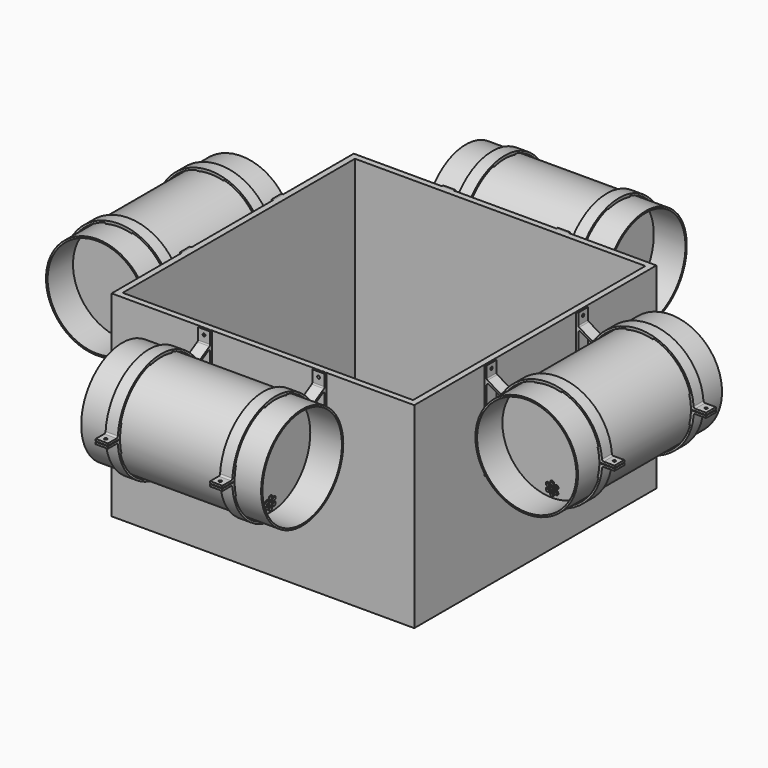
from build123d import *

# Parameters (mm, degrees)
F1_DEPTH    = 139.7
F3_COUNT    = 4
F4_W        = 469.9
F4_H        = 469.9
F4_W_2      = 450.85
F4_H_2      = 450.85
F5_DEPTH    = 304.8
F8_R        = 3.175
F9_DEPTH    = 1.5875
F14_COUNT   = 4
F16_DEPTH   = 9.525
F17_DEPTH   = 9.525
F19_D       = 4.318
F19_DEPTH   = 12.7
F19_TIP     = 1.2972580765
F21_D       = 4.318
F21_DEPTH   = 12.7
F21_TIP     = 1.2972580765
F21_2_D     = 4.318
F21_2_DEPTH = 12.7
F21_2_TIP   = 1.2972580765
F23_COUNT   = 4


with BuildPart() as f1:
    # F0 (on Front) → F1 (new body, symmetric)
    with BuildSketch(Plane.XZ):
        with BuildLine():
            ThreePointArc((413.0675, 228.6), (333.375, 308.2925), (253.6825, 228.6))
            ThreePointArc((253.6825, 228.6), (333.375, 148.9075), (413.0675, 228.6))
        make_face()
        with BuildLine():
            ThreePointArc((410.5275, 228.6), (333.375, 151.4475), (256.2225, 228.6))
            ThreePointArc((256.2225, 228.6), (333.375, 305.7525), (410.5275, 228.6))
        make_face(mode=Mode.SUBTRACT)
    extrude(amount=F1_DEPTH, both=True)


with BuildPart() as f3_1:
    # F3: instance of F1
    add(f1.part.rotate(Axis((0, 0, 60.423810035), (0, 0, 1)), 1 * 360 / F3_COUNT))


with BuildPart() as f3_2:
    # F3: instance of F1
    add(f1.part.rotate(Axis((0, 0, 60.423810035), (0, 0, 1)), 2 * 360 / F3_COUNT))


with BuildPart() as f3_3:
    # F3: instance of F1
    add(f1.part.rotate(Axis((0, 0, 60.423810035), (0, 0, 1)), 3 * 360 / F3_COUNT))


with BuildPart() as f5:
    # F4 (on Top) → F5 (new body)
    with BuildSketch(Plane.XY):
        Rectangle(F4_W, F4_H)
        Rectangle(F4_W_2, F4_H_2, mode=Mode.SUBTRACT)
    extrude(amount=F5_DEPTH)

    # F21 (one way)
    with BuildSketch(Plane.XZ.offset(238.125)):
        with Locations((88.9, 296.855700245), (88.9, 160.344299755)):
            Circle(F21_D / 2)
    extrude(amount=-F21_DEPTH, mode=Mode.SUBTRACT)
    with Locations(Plane.XZ.offset(238.125)):
        with Locations((88.9, 296.855700245), (88.9, 160.344299755)):
            with Locations((0, 0, -(F21_DEPTH + F21_TIP / 2))):  # 118° drill point
                Cone(0, F21_D / 2, F21_TIP, mode=Mode.SUBTRACT)


with BuildPart() as f9:
    # F8 (on Right) → F9 (new body, symmetric)
    with BuildSketch(Plane.YZ):
        with BuildLine():
            ThreePointArc((-333.375, 151.4475), (-278.8199440645, 174.0449440645), (-256.2225, 228.6))
            ThreePointArc((-256.2225, 228.6), (-387.9300559355, 283.1550559355), (-333.375, 151.4475))
        make_face()
        with Locations((-339.9741135768, 160.3375)):
            Circle(F8_R, mode=Mode.SUBTRACT)
        with BuildLine():
            ThreePointArc((-330.2, 156.5275), (-331.1299359697, 154.2824359697), (-333.375, 153.3525))
            ThreePointArc((-333.375, 153.3525), (-336.55, 156.5275), (-333.375, 159.7025))
            ThreePointArc((-333.375, 159.7025), (-331.1299359697, 158.7725640303), (-330.2, 156.5275))
        make_face(mode=Mode.SUBTRACT)
        with BuildLine():
            ThreePointArc((-330.2, 164.1475), (-331.1299359697, 161.9024359697), (-333.375, 160.9725))
            ThreePointArc((-333.375, 160.9725), (-336.55, 164.1475), (-333.375, 167.3225))
            ThreePointArc((-333.375, 167.3225), (-331.1299359697, 166.3925640303), (-330.2, 164.1475))
        make_face(mode=Mode.SUBTRACT)
        with Locations((-339.9741135768, 167.9575)):
            Circle(F8_R, mode=Mode.SUBTRACT)
        with BuildLine():
            ThreePointArc((-330.2, 171.7675), (-331.1299359697, 169.5224359697), (-333.375, 168.5925))
            ThreePointArc((-333.375, 168.5925), (-336.55, 171.7675), (-333.375, 174.9425))
            ThreePointArc((-333.375, 174.9425), (-331.1299359697, 174.0125640303), (-330.2, 171.7675))
        make_face(mode=Mode.SUBTRACT)
        with Locations((-326.7758864232, 160.3375)):
            Circle(F8_R, mode=Mode.SUBTRACT)
        with Locations((-326.7758864232, 167.9575)):
            Circle(F8_R, mode=Mode.SUBTRACT)
    extrude(amount=F9_DEPTH, both=True)


with BuildPart() as f12_1:
    # F12: instance of F9
    add(f9.part.mirror(Plane.YZ.offset(-44.45)))


with BuildPart() as f13_1:
    # F13: instance of F9
    add(f9.part.mirror(Plane.YZ.offset(44.45)))


with BuildPart() as f14_1:
    # F14: instance of F13_1
    add(f13_1.part.rotate(Axis((0, 0, 60.423810035), (0, 0, 1)), 1 * 360 / F14_COUNT))


with BuildPart() as f14_2:
    # F14: instance of F13_1
    add(f13_1.part.rotate(Axis((0, 0, 60.423810035), (0, 0, 1)), 2 * 360 / F14_COUNT))


with BuildPart() as f14_3:
    # F14: instance of F13_1
    add(f13_1.part.rotate(Axis((0, 0, 60.423810035), (0, 0, 1)), 3 * 360 / F14_COUNT))


with BuildPart() as f14_4:
    # F14: instance of F12_1
    add(f12_1.part.rotate(Axis((0, 0, 60.423810035), (0, 0, 1)), 1 * 360 / F14_COUNT))


with BuildPart() as f14_5:
    # F14: instance of F12_1
    add(f12_1.part.rotate(Axis((0, 0, 60.423810035), (0, 0, 1)), 2 * 360 / F14_COUNT))


with BuildPart() as f14_6:
    # F14: instance of F12_1
    add(f12_1.part.rotate(Axis((0, 0, 60.423810035), (0, 0, 1)), 3 * 360 / F14_COUNT))


with BuildPart() as f14_7:
    # F14: instance of F9
    add(f9.part.rotate(Axis((0, 0, 60.423810035), (0, 0, 1)), 1 * 360 / F14_COUNT))


with BuildPart() as f14_8:
    # F14: instance of F9
    add(f9.part.rotate(Axis((0, 0, 60.423810035), (0, 0, 1)), 2 * 360 / F14_COUNT))


with BuildPart() as f14_9:
    # F14: instance of F9
    add(f9.part.rotate(Axis((0, 0, 60.423810035), (0, 0, 1)), 3 * 360 / F14_COUNT))


with BuildPart() as f16:
    # F15 (on offset) → F16 (new body, symmetric)
    with BuildSketch(Plane.YZ.offset(88.9)):
        Polygon((-234.15625, 284.0508849165), (-234.95, 285.425700245), (-234.95, 283.5926131403), align=None)
        Polygon((-234.95, 173.6073868597), (-234.95, 171.774299755), (-234.15625, 173.1491150835), align=None)
        with BuildLine():
            Line((-234.95, 171.774299755), (-260.5097875891, 186.53125))
            ThreePointArc((-260.5097875891, 186.53125), (-261.5323767442, 184.8078044626), (-262.5957219044, 183.1092020457))
            ThreePointArc((-262.5957219044, 183.1092020457), (-261.0577707968, 184.2043074512), (-259.1889889808, 183.9355994633))
            Line((-259.1889889808, 183.9355994633), (-239.395, 172.5075345969))
            ThreePointArc((-239.395, 172.5075345969), (-238.4652954744, 171.5778300713), (-238.125, 170.3078300713))
            Line((-238.125, 170.3078300713), (-238.125, 152.724299755))
            Line((-238.125, 152.724299755), (-234.95, 152.724299755))
            Line((-234.95, 152.724299755), (-234.95, 171.774299755))
        make_face()
        with BuildLine():
            Line((-234.95, 228.6), (-249.2375, 228.6))
            ThreePointArc((-249.2375, 228.6), (-249.2613654173, 226.596157805), (-249.3329481306, 224.593452381))
            ThreePointArc((-249.3329481306, 224.593452381), (-248.5485961043, 226.3108170357), (-246.7958295836, 227.0125))
            Line((-246.7958295836, 227.0125), (-240.665, 227.0125))
            ThreePointArc((-240.665, 227.0125), (-238.8689487758, 226.2685512242), (-238.125, 224.4725))
            Line((-238.125, 224.4725), (-238.125, 179.8398830156))
            ThreePointArc((-238.125, 179.8398830156), (-239.395, 177.64017849), (-241.935, 177.64017849))
            Line((-241.935, 177.64017849), (-257.6014889808, 186.6852301203))
            ThreePointArc((-257.6014889808, 186.6852301203), (-258.7685878325, 188.1692886531), (-258.5891742854, 190.0487460848))
            ThreePointArc((-258.5891742854, 190.0487460848), (-259.5285345493, 188.2785609547), (-260.5097875891, 186.53125))
            Line((-260.5097875891, 186.53125), (-234.95, 171.774299755))
            Line((-234.95, 171.774299755), (-234.95, 173.6073868597))
            Line((-234.95, 173.6073868597), (-234.95, 227.0125))
            Line((-234.95, 227.0125), (-234.95, 228.6))
        make_face()
        with BuildLine():
            ThreePointArc((-312.3381880141, 307.1104511608), (-283.8948710502, 293.0837594989), (-262.9844551804, 269.24))
            Line((-262.9844551804, 269.24), (-260.5097875891, 270.66875))
            Line((-260.5097875891, 270.66875), (-234.95, 285.425700245))
            Line((-234.95, 285.425700245), (-234.95, 304.475700245))
            Line((-234.95, 304.475700245), (-238.125, 304.475700245))
            Line((-238.125, 304.475700245), (-238.125, 286.8921699287))
            ThreePointArc((-238.125, 286.8921699287), (-238.4652954744, 285.6221699287), (-239.395, 284.6924654031))
            Line((-239.395, 284.6924654031), (-259.1889889808, 273.2644005367))
            ThreePointArc((-259.1889889808, 273.2644005367), (-261.0577707968, 272.9956925488), (-262.5957219044, 274.0907979543))
            ThreePointArc((-262.5957219044, 274.0907979543), (-354.1656429935, 310.1283267961), (-417.2953763233, 234.6406410256))
            ThreePointArc((-417.2953763233, 234.6406410256), (-418.0984447791, 232.9635925951), (-419.8288216463, 232.283))
            Line((-419.8288216463, 232.283), (-436.5625, 232.283))
            Line((-436.5625, 232.283), (-436.5625, 229.108))
            Line((-436.5625, 229.108), (-417.5109664011, 229.108))
            Line((-417.5109664011, 229.108), (-414.6534124845, 229.108))
            ThreePointArc((-414.6534124845, 229.108), (-413.9260910333, 239.4609453249), (-411.8854511608, 249.6368119859))
            ThreePointArc((-411.8854511608, 249.6368119859), (-390.8486391748, 286.0736391748), (-354.4118119859, 307.1104511608))
            ThreePointArc((-354.4118119859, 307.1104511608), (-343.9841689036, 309.1846383325), (-333.375, 309.88))
            ThreePointArc((-333.375, 309.88), (-322.7658310964, 309.1846383325), (-312.3381880141, 307.1104511608))
        make_face()
        with BuildLine():
            Line((-260.5097875891, 186.53125), (-262.9844551804, 187.96))
            ThreePointArc((-262.9844551804, 187.96), (-283.8948710502, 164.1162405011), (-312.3381880141, 150.0895488392))
            ThreePointArc((-312.3381880141, 150.0895488392), (-333.375, 147.32), (-354.4118119859, 150.0895488392))
            ThreePointArc((-354.4118119859, 150.0895488392), (-390.8486391748, 171.1263608252), (-411.8854511608, 207.5631880141))
            ThreePointArc((-411.8854511608, 207.5631880141), (-413.9260910333, 217.7390546751), (-414.6534124845, 228.092))
            Line((-414.6534124845, 228.092), (-417.5109664011, 228.092))
            Line((-417.5109664011, 228.092), (-436.5625, 228.092))
            Line((-436.5625, 228.092), (-436.5625, 224.917))
            Line((-436.5625, 224.917), (-419.8288216463, 224.917))
            ThreePointArc((-419.8288216463, 224.917), (-418.0984447791, 224.2364074049), (-417.2953763233, 222.5593589744))
            ThreePointArc((-417.2953763233, 222.5593589744), (-354.1656429935, 147.0716732039), (-262.5957219044, 183.1092020457))
            ThreePointArc((-262.5957219044, 183.1092020457), (-261.5323767442, 184.8078044626), (-260.5097875891, 186.53125))
        make_face()
        with BuildLine():
            ThreePointArc((-254.8645488392, 249.6368119859), (-252.7903616675, 239.2091689036), (-252.095, 228.6))
            Line((-252.095, 228.6), (-249.2375, 228.6))
            Line((-249.2375, 228.6), (-234.95, 228.6))
            Line((-234.95, 228.6), (-234.95, 230.1875))
            Line((-234.95, 230.1875), (-234.95, 283.5926131403))
            Line((-234.95, 283.5926131403), (-234.95, 285.425700245))
            Line((-234.95, 285.425700245), (-260.5097875891, 270.66875))
            Line((-260.5097875891, 270.66875), (-262.9844551804, 269.24))
            ThreePointArc((-262.9844551804, 269.24), (-258.2820715975, 259.7045093826), (-254.8645488392, 249.6368119859))
        make_face()
        with BuildLine():
            ThreePointArc((-238.125, 232.7275), (-238.8689487758, 230.9314487758), (-240.665, 230.1875))
            Line((-240.665, 230.1875), (-246.7958295836, 230.1875))
            ThreePointArc((-246.7958295836, 230.1875), (-248.5485961043, 230.8891829643), (-249.3329481306, 232.606547619))
            ThreePointArc((-249.3329481306, 232.606547619), (-252.1044157906, 250.3763874073), (-258.5891742854, 267.1512539152))
            ThreePointArc((-258.5891742854, 267.1512539152), (-258.7685878325, 269.0307113469), (-257.6014889808, 270.5147698797))
            Line((-257.6014889808, 270.5147698797), (-241.935, 279.55982151))
            ThreePointArc((-241.935, 279.55982151), (-239.395, 279.55982151), (-238.125, 277.3601169844))
            Line((-238.125, 277.3601169844), (-238.125, 232.7275))
        make_face(mode=Mode.SUBTRACT)
        with BuildLine():
            Line((-249.2375, 228.6), (-252.095, 228.6))
            ThreePointArc((-252.095, 228.6), (-252.7903616675, 217.9908310964), (-254.8645488392, 207.5631880141))
            ThreePointArc((-254.8645488392, 207.5631880141), (-258.2820715975, 197.4954906174), (-262.9844551804, 187.96))
            Line((-262.9844551804, 187.96), (-260.5097875891, 186.53125))
            ThreePointArc((-260.5097875891, 186.53125), (-259.5285345493, 188.2785609547), (-258.5891742854, 190.0487460848))
            ThreePointArc((-258.5891742854, 190.0487460848), (-252.1044157906, 206.8236125927), (-249.3329481306, 224.593452381))
            ThreePointArc((-249.3329481306, 224.593452381), (-249.2613654173, 226.596157805), (-249.2375, 228.6))
        make_face()
    extrude(amount=F16_DEPTH, both=True)

    # F19
    with Locations(Plane.XY.offset(232.283)):
        with Locations((88.9, -428.9425)):
            Hole(F19_D / 2, depth=F19_DEPTH)
            with Locations((0, 0, -(F19_DEPTH + F19_TIP / 2))):  # 118° drill point
                Cone(0, F19_D / 2, F19_TIP, mode=Mode.SUBTRACT)

    # F21#2 (one way)
    with BuildSketch(Plane.XZ.offset(238.125)):
        with Locations((88.9, 296.855700245), (88.9, 160.344299755)):
            Circle(F21_2_D / 2)
    extrude(amount=-F21_2_DEPTH, mode=Mode.SUBTRACT)
    with Locations(Plane.XZ.offset(238.125)):
        with Locations((88.9, 296.855700245), (88.9, 160.344299755)):
            with Locations((0, 0, -(F21_2_DEPTH + F21_2_TIP / 2))):  # 118° drill point
                Cone(0, F21_2_D / 2, F21_2_TIP, mode=Mode.SUBTRACT)


with BuildPart() as f17:
    # F15 (on offset) → F17 (new body, symmetric)
    with BuildSketch(Plane.YZ.offset(88.9)):
        with BuildLine():
            Line((-253.6825, 228.6), (-252.095, 228.6))
            ThreePointArc((-252.095, 228.6), (-252.7903616675, 239.2091689036), (-254.8645488392, 249.6368119859))
            Line((-254.8645488392, 249.6368119859), (-256.3979560885, 249.2259367518))
            ThreePointArc((-256.3979560885, 249.2259367518), (-254.364280385, 239.0019585735), (-253.6825, 228.6))
        make_face()
        with BuildLine():
            ThreePointArc((-254.8645488392, 207.5631880141), (-252.7903616675, 217.9908310964), (-252.095, 228.6))
            Line((-252.095, 228.6), (-253.6825, 228.6))
            ThreePointArc((-253.6825, 228.6), (-254.364280385, 218.1980414265), (-256.3979560885, 207.9740632482))
            Line((-256.3979560885, 207.9740632482), (-254.8645488392, 207.5631880141))
        make_face()
    extrude(amount=F17_DEPTH, both=True)


with BuildPart() as f17b:
    # F15 (on offset) → F17, piece 2 (new body, symmetric)
    with BuildSketch(Plane.YZ.offset(88.9)):
        with BuildLine():
            Line((-312.7490632482, 305.5770439115), (-312.3381880141, 307.1104511608))
            ThreePointArc((-312.3381880141, 307.1104511608), (-322.7658310964, 309.1846383325), (-333.375, 309.88))
            Line((-333.375, 309.88), (-333.375, 308.2925))
            ThreePointArc((-333.375, 308.2925), (-322.9730414265, 307.610719615), (-312.7490632482, 305.5770439115))
        make_face()
        with BuildLine():
            ThreePointArc((-354.0009367518, 305.5770439115), (-343.7769585735, 307.610719615), (-333.375, 308.2925))
            Line((-333.375, 308.2925), (-333.375, 309.88))
            ThreePointArc((-333.375, 309.88), (-343.9841689036, 309.1846383325), (-354.4118119859, 307.1104511608))
            Line((-354.4118119859, 307.1104511608), (-354.0009367518, 305.5770439115))
        make_face()
    extrude(amount=F17_DEPTH, both=True)


with BuildPart() as f17c:
    # F15 (on offset) → F17, piece 3 (new body, symmetric)
    with BuildSketch(Plane.YZ.offset(88.9)):
        with BuildLine():
            ThreePointArc((-354.4118119859, 150.0895488392), (-333.375, 147.32), (-312.3381880141, 150.0895488392))
            Line((-312.3381880141, 150.0895488392), (-312.7490632482, 151.6229560885))
            ThreePointArc((-312.7490632482, 151.6229560885), (-333.375, 148.9075), (-354.0009367518, 151.6229560885))
            Line((-354.0009367518, 151.6229560885), (-354.4118119859, 150.0895488392))
        make_face()
    extrude(amount=F17_DEPTH, both=True)


with BuildPart() as f17d:
    # F15 (on offset) → F17, piece 4 (new body, symmetric)
    with BuildSketch(Plane.YZ.offset(88.9)):
        with BuildLine():
            ThreePointArc((-410.3520439115, 207.9740632482), (-413.0675, 228.6), (-410.3520439115, 249.2259367518))
            Line((-410.3520439115, 249.2259367518), (-411.8854511608, 249.6368119859))
            ThreePointArc((-411.8854511608, 249.6368119859), (-413.9260910333, 239.4609453249), (-414.6534124845, 229.108))
            ThreePointArc((-414.6534124845, 229.108), (-414.6546031202, 228.8540012403), (-414.655, 228.6))
            ThreePointArc((-414.655, 228.6), (-414.6546031202, 228.3459987597), (-414.6534124845, 228.092))
            ThreePointArc((-414.6534124845, 228.092), (-413.9260910333, 217.7390546751), (-411.8854511608, 207.5631880141))
            Line((-411.8854511608, 207.5631880141), (-410.3520439115, 207.9740632482))
        make_face()
    extrude(amount=F17_DEPTH, both=True)


with BuildPart() as f22_1:
    # F22: instance of F17c
    add(f17c.part.mirror(Plane.YZ))


with BuildPart() as f22_2:
    # F22: instance of F17d
    add(f17d.part.mirror(Plane.YZ))


with BuildPart() as f22_3:
    # F22: instance of F17b
    add(f17b.part.mirror(Plane.YZ))


with BuildPart() as f22_4:
    # F22: instance of F17
    add(f17.part.mirror(Plane.YZ))


with BuildPart() as f22_5:
    # F22: instance of F16
    add(f16.part.mirror(Plane.YZ))


with BuildPart() as f23_1:
    # F23: instance of F22_1
    add(f22_1.part.rotate(Axis((0, 0, 60.423810035), (0, 0, 1)), 1 * 360 / F23_COUNT))


with BuildPart() as f23_2:
    # F23: instance of F22_1
    add(f22_1.part.rotate(Axis((0, 0, 60.423810035), (0, 0, 1)), 2 * 360 / F23_COUNT))


with BuildPart() as f23_3:
    # F23: instance of F22_1
    add(f22_1.part.rotate(Axis((0, 0, 60.423810035), (0, 0, 1)), 3 * 360 / F23_COUNT))


with BuildPart() as f23_4:
    # F23: instance of F22_2
    add(f22_2.part.rotate(Axis((0, 0, 60.423810035), (0, 0, 1)), 1 * 360 / F23_COUNT))


with BuildPart() as f23_5:
    # F23: instance of F22_2
    add(f22_2.part.rotate(Axis((0, 0, 60.423810035), (0, 0, 1)), 2 * 360 / F23_COUNT))


with BuildPart() as f23_6:
    # F23: instance of F22_2
    add(f22_2.part.rotate(Axis((0, 0, 60.423810035), (0, 0, 1)), 3 * 360 / F23_COUNT))


with BuildPart() as f23_7:
    # F23: instance of F22_3
    add(f22_3.part.rotate(Axis((0, 0, 60.423810035), (0, 0, 1)), 1 * 360 / F23_COUNT))


with BuildPart() as f23_8:
    # F23: instance of F22_3
    add(f22_3.part.rotate(Axis((0, 0, 60.423810035), (0, 0, 1)), 2 * 360 / F23_COUNT))


with BuildPart() as f23_9:
    # F23: instance of F22_3
    add(f22_3.part.rotate(Axis((0, 0, 60.423810035), (0, 0, 1)), 3 * 360 / F23_COUNT))


with BuildPart() as f23_10:
    # F23: instance of F22_4
    add(f22_4.part.rotate(Axis((0, 0, 60.423810035), (0, 0, 1)), 1 * 360 / F23_COUNT))


with BuildPart() as f23_11:
    # F23: instance of F22_4
    add(f22_4.part.rotate(Axis((0, 0, 60.423810035), (0, 0, 1)), 2 * 360 / F23_COUNT))


with BuildPart() as f23_12:
    # F23: instance of F22_4
    add(f22_4.part.rotate(Axis((0, 0, 60.423810035), (0, 0, 1)), 3 * 360 / F23_COUNT))


with BuildPart() as f23_13:
    # F23: instance of F22_5
    add(f22_5.part.rotate(Axis((0, 0, 60.423810035), (0, 0, 1)), 1 * 360 / F23_COUNT))


with BuildPart() as f23_14:
    # F23: instance of F22_5
    add(f22_5.part.rotate(Axis((0, 0, 60.423810035), (0, 0, 1)), 2 * 360 / F23_COUNT))


with BuildPart() as f23_15:
    # F23: instance of F22_5
    add(f22_5.part.rotate(Axis((0, 0, 60.423810035), (0, 0, 1)), 3 * 360 / F23_COUNT))


with BuildPart() as f23_16:
    # F23: instance of F17c
    add(f17c.part.rotate(Axis((0, 0, 60.423810035), (0, 0, 1)), 1 * 360 / F23_COUNT))


with BuildPart() as f23_17:
    # F23: instance of F17c
    add(f17c.part.rotate(Axis((0, 0, 60.423810035), (0, 0, 1)), 2 * 360 / F23_COUNT))


with BuildPart() as f23_18:
    # F23: instance of F17c
    add(f17c.part.rotate(Axis((0, 0, 60.423810035), (0, 0, 1)), 3 * 360 / F23_COUNT))


with BuildPart() as f23_19:
    # F23: instance of F17d
    add(f17d.part.rotate(Axis((0, 0, 60.423810035), (0, 0, 1)), 1 * 360 / F23_COUNT))


with BuildPart() as f23_20:
    # F23: instance of F17d
    add(f17d.part.rotate(Axis((0, 0, 60.423810035), (0, 0, 1)), 2 * 360 / F23_COUNT))


with BuildPart() as f23_21:
    # F23: instance of F17d
    add(f17d.part.rotate(Axis((0, 0, 60.423810035), (0, 0, 1)), 3 * 360 / F23_COUNT))


with BuildPart() as f23_22:
    # F23: instance of F17b
    add(f17b.part.rotate(Axis((0, 0, 60.423810035), (0, 0, 1)), 1 * 360 / F23_COUNT))


with BuildPart() as f23_23:
    # F23: instance of F17b
    add(f17b.part.rotate(Axis((0, 0, 60.423810035), (0, 0, 1)), 2 * 360 / F23_COUNT))


with BuildPart() as f23_24:
    # F23: instance of F17b
    add(f17b.part.rotate(Axis((0, 0, 60.423810035), (0, 0, 1)), 3 * 360 / F23_COUNT))


with BuildPart() as f23_25:
    # F23: instance of F17
    add(f17.part.rotate(Axis((0, 0, 60.423810035), (0, 0, 1)), 1 * 360 / F23_COUNT))


with BuildPart() as f23_26:
    # F23: instance of F17
    add(f17.part.rotate(Axis((0, 0, 60.423810035), (0, 0, 1)), 2 * 360 / F23_COUNT))


with BuildPart() as f23_27:
    # F23: instance of F17
    add(f17.part.rotate(Axis((0, 0, 60.423810035), (0, 0, 1)), 3 * 360 / F23_COUNT))


with BuildPart() as f23_28:
    # F23: instance of F16
    add(f16.part.rotate(Axis((0, 0, 60.423810035), (0, 0, 1)), 1 * 360 / F23_COUNT))


with BuildPart() as f23_29:
    # F23: instance of F16
    add(f16.part.rotate(Axis((0, 0, 60.423810035), (0, 0, 1)), 2 * 360 / F23_COUNT))


with BuildPart() as f23_30:
    # F23: instance of F16
    add(f16.part.rotate(Axis((0, 0, 60.423810035), (0, 0, 1)), 3 * 360 / F23_COUNT))


solid = Compound([f1.part, f3_1.part, f3_2.part, f3_3.part, f5.part, f9.part, f12_1.part, f13_1.part, f14_1.part, f14_2.part, f14_3.part, f14_4.part, f14_5.part, f14_6.part, f14_7.part, f14_8.part, f14_9.part, f16.part, f17.part, f17b.part, f17c.part, f17d.part, f22_1.part, f22_2.part, f22_3.part, f22_4.part, f22_5.part, f23_1.part, f23_2.part, f23_3.part, f23_4.part, f23_5.part, f23_6.part, f23_7.part, f23_8.part, f23_9.part, f23_10.part, f23_11.part, f23_12.part, f23_13.part, f23_14.part, f23_15.part, f23_16.part, f23_17.part, f23_18.part, f23_19.part, f23_20.part, f23_21.part, f23_22.part, f23_23.part, f23_24.part, f23_25.part, f23_26.part, f23_27.part, f23_28.part, f23_29.part, f23_30.part])
